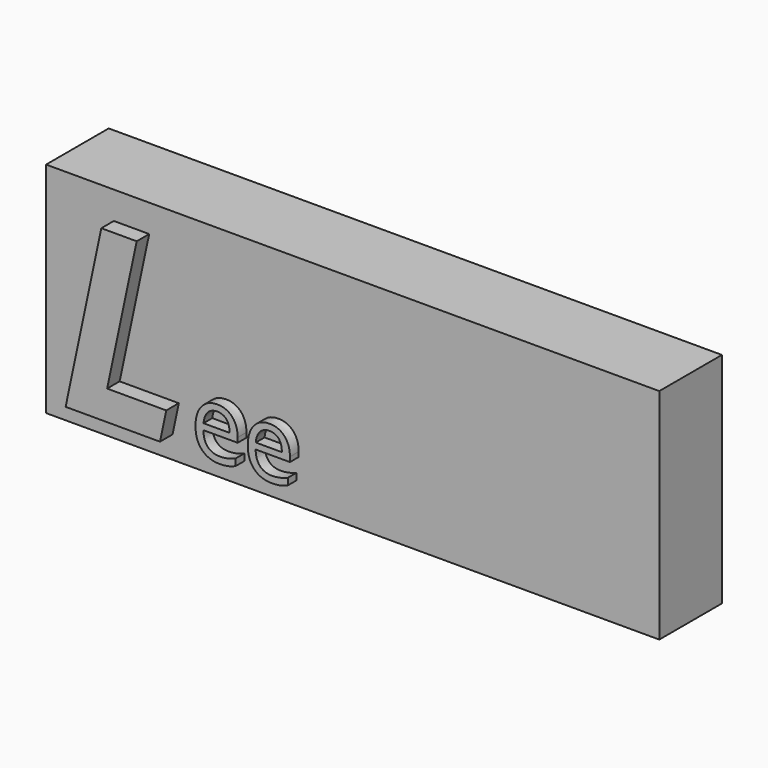
from build123d import *

# Parameters (mm, degrees)
F0_W         = 99.4594395161
F0_H         = 35.488307476
F1_DEPTH     = 12.7
F2_TEXT_SIZE = 38.3663169082
F3_DEPTH     = 2.54
F4_TEXT_SIZE = 15.1068551026
F5_DEPTH     = 1.778


# Not quite as in the source:
# - Text() gives the source's letters only with a copy of the font that has no kerning and outlines rounded to 1/6400 em; it was checked with that copy


with BuildPart() as f1:
    # F0 (on Front) → F1 (new body)
    with BuildSketch(Plane.XZ):
        with Locations((49.729719758, 17.744153738)):
            Rectangle(F0_W, F0_H)
    extrude(amount=F1_DEPTH)

    # F2 (on face) → F3 (join)
    with BuildSketch(Plane.XZ.offset(12.7)):
        with Locations((4.2084991001, 3.6166498903)):
            Text('L', F2_TEXT_SIZE, font='Open Sans', font_style=FontStyle.BOLDITALIC, text_align=(TextAlign.LEFT, TextAlign.BOTTOM))
    extrude(amount=F3_DEPTH)

    # F4 (on face) → F5 (join)
    with BuildSketch(Plane.XZ.offset(12.7)):
        with Locations((24.8110909015, 3.2262096647)):
            Text('ee', F4_TEXT_SIZE, font='Open Sans', text_align=(TextAlign.LEFT, TextAlign.BOTTOM))
    extrude(amount=F5_DEPTH)


solid = f1.part
